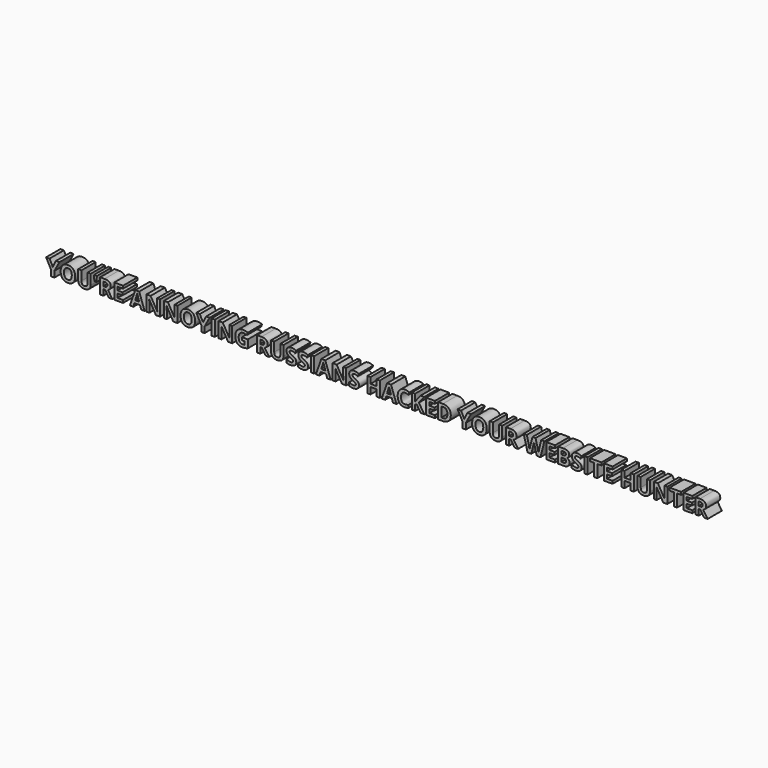
from build123d import *

# Parameters (mm, degrees)
F0_TEXT_SIZE = 132.2980711444
F1_DEPTH     = 110.49


# Not quite as in the source:
# - Text() gives the source's letters only with a copy of the font that has no kerning and outlines rounded to 1/6400 em; it was checked with that copy


with BuildPart() as f1:
    # F0 (on Front) → F1 (new body)
    with BuildSketch(Plane.XZ):
        with Locations((-110.1652830839, -61.6781301796)):
            Text("YOU'RE ANNOYING RUSSIANS HACKED YOUR WEBSITE HUNTER", F0_TEXT_SIZE, font='Open Sans', font_style=FontStyle.BOLD, text_align=(TextAlign.LEFT, TextAlign.BOTTOM))
    extrude(amount=F1_DEPTH)


solid = f1.part
